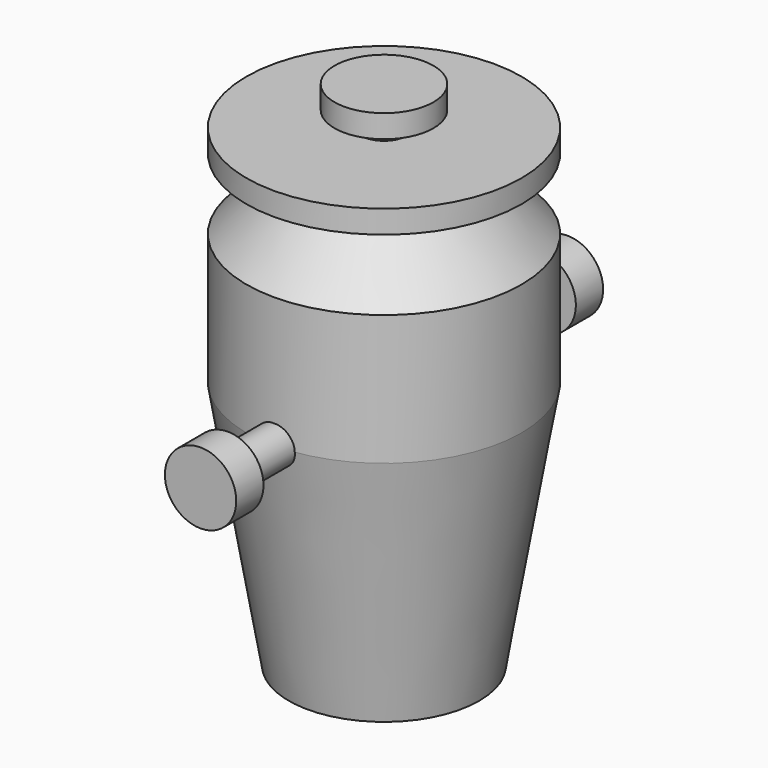
from build123d import *


with BuildPart() as f1:
    # F0 (on Front) → F1 (revolve)
    with BuildSketch(Plane.XZ):
        Polygon((0, 171.6705819281), (0, 0), (0, -163.3294180719), (62.310040211, -163.3294180719), (90, 0), (90, 85.3906134428), (58.0335408158, 121.6705819281), (58.0335408158, 131.6705819281), (90, 131.6705819281), (90, 146.6705819281), (15, 146.6705819281), (15, 156.6705819281), (32.3543744587, 156.6705819281), (32.3543744587, 171.6705819281), align=None)
    revolve(axis=Axis((0, 0, 85.8352909641), (0, 0, 1)))


with BuildPart() as f3:
    # F2 (on Right) → F3 (revolve)
    with BuildSketch(Plane.YZ):
        Polygon((0, -12.8155195192), (0, 0), (-127.7133935073, 0), (-150, 0), (-150, -23.3408341183), (-127.7133935073, -23.3408341183), (-127.7133935073, -12.8155195192), align=None)
    revolve(axis=Axis((0, -63.8566967536, 0), (0, -1, 0)))

    # F4: F3 across plane


with BuildPart() as f3_1:
    add(f3.part)
    add(f3.part.mirror(Plane.XZ))


solid = Compound([f1.part, f3_1.part])
